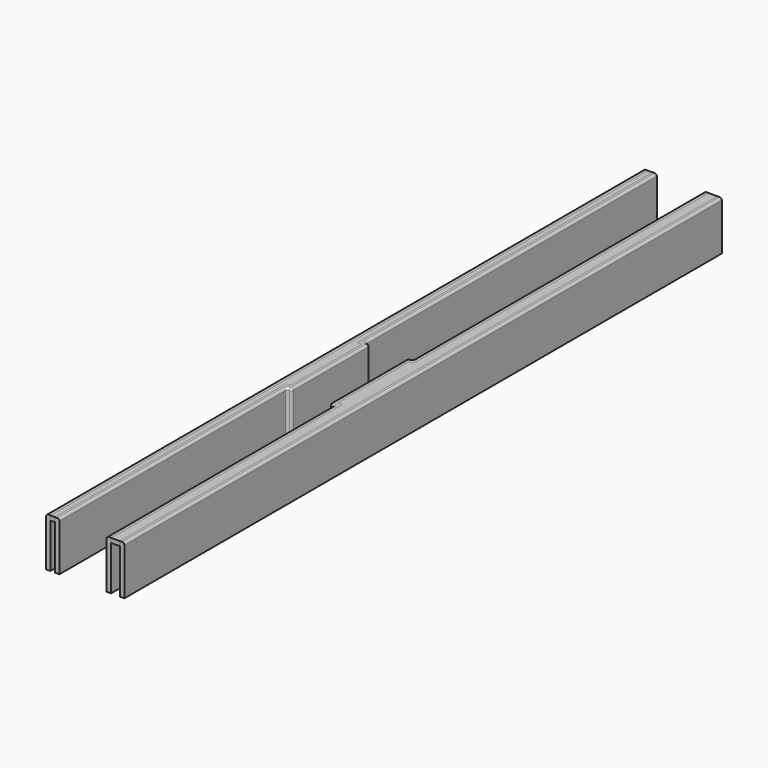
from build123d import *

# Parameters (mm, degrees)
F0_W     = 1
F0_H     = 20
F1_DEPTH = 1
F0_H_2   = 168
F2_DEPTH = 11
F3_R     = 0.49999
F3_2_R   = 0.49999
F3_3_R   = 0.49999
F3_4_R   = 0.49999


# Not quite as in the source:
# - a fillet or chamfer is up to 0.001 mm smaller than in the source, because OpenCascade refuses the exact size


with BuildPart() as f1:
    # F0 (on Top) → F1 (new body)
    with BuildSketch(Plane.XY):
        Polygon((-1, 0), (0, 0), (0, 65), (0, 85), (0, 168), (-1, 168), align=None)
        with Locations((0.5, 75)):
            Rectangle(F0_W, F0_H)
    extrude(amount=-F1_DEPTH)


with BuildPart() as f1b:
    # F0 (on Top) → F1, piece 2 (new body)
    with BuildSketch(Plane.XY):
        Polygon((12.6243081391, 65), (12.6243081391, 0), (14.6243081391, 0), (14.6243081391, 168), (12.6243081391, 168), (12.6243081391, 85), align=None)
        with Locations((12.1243081391, 75)):
            Rectangle(F0_W, F0_H)
    extrude(amount=-F1_DEPTH)


with BuildPart() as f2:
    # F0 (on Top) → F2 (new body)
    with BuildSketch(Plane.XY):
        with Locations((-1.5, 84)):
            Rectangle(F0_W, F0_H_2)
    extrude(amount=-F2_DEPTH)

    # F3#4 (radius 0.5 in the source; OpenCascade refuses exactly that, so slightly less here)
    f3_4_edges = [f2.edges().sort_by_distance(p)[0] for p in [
        (-2, 84, 0),
    ]]
    fillet(f3_4_edges, radius=F3_4_R)


with BuildPart() as f2b:
    # F0 (on Top) → F2, piece 2 (new body)
    with BuildSketch(Plane.XY):
        Polygon((0, 168), (0, 85), (1, 85), (1, 86), (1, 168), align=None)
        Polygon((1, 85), (1, 65), (1, 64), (2, 64), (2, 86), (1, 86), align=None)
        Polygon((0, 65), (0, 0), (1, 0), (1, 64), (1, 65), align=None)
    extrude(amount=-F2_DEPTH)

    # F3#3 (radius 0.5 in the source; OpenCascade refuses exactly that, so slightly less here)
    f3_3_edges = [f2b.edges().sort_by_distance(p)[0] for p in [
        (1, 32, 0),
        (2, 75, 0),
        (1, 127, 0),
        (1.5, 86, 0),
        (1.5, 64, 0),
        (2, 64, -5.5),
        (2, 86, -5.5),
        (1, 86, -5.5),
        (1, 64, -5.5),
    ]]
    fillet(f3_3_edges, radius=F3_3_R)


with BuildPart() as f2c:
    # F0 (on Top) → F2, piece 3 (new body)
    with BuildSketch(Plane.XY):
        Polygon((11.6243081391, 64), (11.6243081391, 65), (11.6243081391, 85), (11.6243081391, 86), (10.6243081391, 86), (10.6243081391, 64), align=None)
        Polygon((11.6243081391, 0), (12.6243081391, 0), (12.6243081391, 65), (11.6243081391, 65), (11.6243081391, 64), align=None)
        Polygon((11.6243081391, 85), (12.6243081391, 85), (12.6243081391, 168), (11.6243081391, 168), (11.6243081391, 86), align=None)
    extrude(amount=-F2_DEPTH)

    # F3#2 (radius 0.5 in the source; OpenCascade refuses exactly that, so slightly less here)
    f3_2_edges = [f2c.edges().sort_by_distance(p)[0] for p in [
        (11.624308, 32, 0),
        (10.624308, 75, 0),
        (11.624308, 127, 0),
        (11.124308, 86, 0),
        (11.124308, 64, 0),
        (10.624308, 64, -5.5),
        (10.624308, 86, -5.5),
        (11.624308, 86, -5.5),
        (11.624308, 64, -5.5),
    ]]
    fillet(f3_2_edges, radius=F3_2_R)


with BuildPart() as f2d:
    # F0 (on Top) → F2, piece 4 (new body)
    with BuildSketch(Plane.XY):
        with Locations((15.1243081391, 84)):
            Rectangle(F0_W, F0_H_2)
    extrude(amount=-F2_DEPTH)

    # F3 (radius 0.5 in the source; OpenCascade refuses exactly that, so slightly less here)
    f3_edges = [f2d.edges().sort_by_distance(p)[0] for p in [
        (15.624308, 84, 0),
    ]]
    fillet(f3_edges, radius=F3_R)


solid = Compound([f1.part, f1b.part, f2.part, f2b.part, f2c.part, f2d.part])
